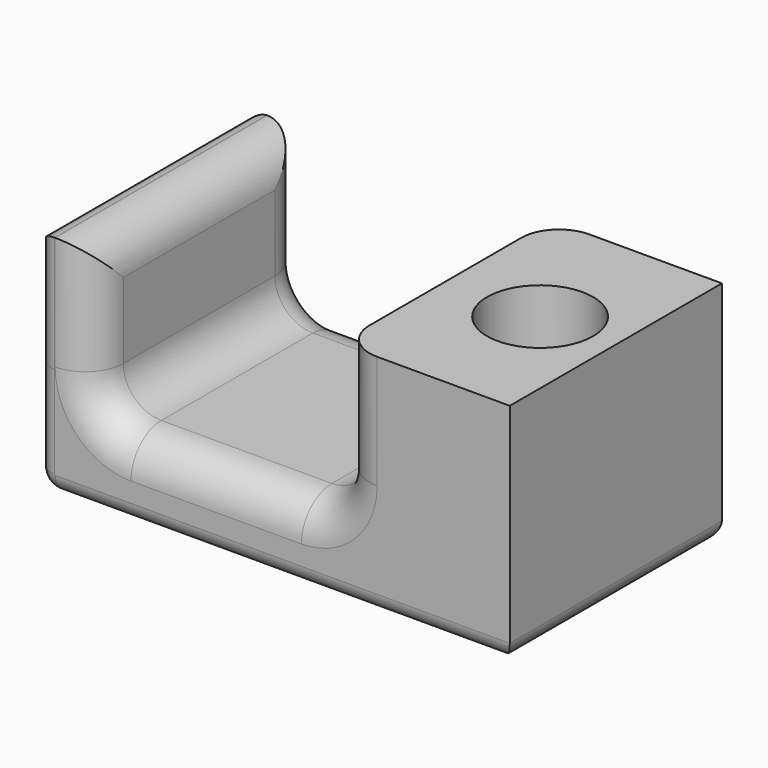
from build123d import *

# Parameters (mm, degrees)
F0_W         = 1.5
F0_H         = 7
F0_W_2       = 6.5
F0_W_3       = 4.5
F0_R         = 1.4
F1_DEPTH     = 2
F2_DEPTH     = 4
F3_F1_R      = 1
F3_F2_R      = 1
F4_T1_DEPTH  = 5.9980686292
F4_T3_DEPTH  = 13.2514489274
F4_T5_DEPTH  = 9.5048292256
F4_T7_DEPTH  = 2.4368940733
F4_T9_DEPTH  = 4.3169803418
F4_T11_DEPTH = 9.509680201
F4_T13_DEPTH = 4.2548401974
F4_T15_DEPTH = 2.4990342177
F4_S19_W     = 0.551502254
F4_S19_H     = 0.5515022539
F4_T20_DEPTH = 0.551502254
F4_S25_W     = 0.551502254
F4_S25_H     = 0.5515022539
F4_T26_DEPTH = 0.551502254


# Not quite as in the source:
# - a fillet or chamfer that OpenCascade refuses, or shapes differently, is made with other operations: its cross-section is extruded or revolved along the edge and cut away or added


with BuildPart() as f1:
    # F0 (on Top) → F1 (new body)
    with BuildSketch(Plane.XY):
        with Locations((-7.4809225276, 0.9873391916)):
            Rectangle(F0_W, F0_H)
        with Locations((-3.4809225276, 0.9873391916)):
            Rectangle(F0_W_2, F0_H)
        with Locations((2.0190774724, 0.9873391916)):
            Rectangle(F0_W_3, F0_H)
        with Locations((2.2690774724, 0.9873391916)):
            Circle(F0_R, mode=Mode.SUBTRACT)
    extrude(amount=-F1_DEPTH)

    # F0 (on Top) → F2 (join)
    with BuildSketch(Plane.XY):
        with Locations((-7.4809225276, 0.9873391916)):
            Rectangle(F0_W, F0_H)
        with Locations((2.0190774724, 0.9873391916)):
            Rectangle(F0_W_3, F0_H)
        with Locations((2.2690774724, 0.9873391916)):
            Circle(F0_R, mode=Mode.SUBTRACT)
    extrude(amount=F2_DEPTH)

    # F3: fillet of radius 1 on 7 edges, made by hand

    # F3_f1
    f3_f1_edges = [f1.edges().sort_by_distance(p)[0] for p in [
        (-0.2309225276, 0.9873391916, 0),
        (-6.7309225276, 0.9873391916, 0),
    ]]
    fillet(f3_f1_edges, radius=F3_F1_R)

    # F3_f2
    f3_f2_edges = [f1.edges().sort_by_distance(p)[0] for p in [
        (-3.4809225276, 4.4873391916, 0),
        (-3.4809225276, -2.5126608084, 0),
        (-6.7309225276, -2.5126608084, 2.5),
        (-6.7309225276, 4.4873391916, 2.5),
        (-6.7309225276, 0.9873391916, 4),
        (-6.4380293088, 4.4873391916, 0.2928932188),
        (-6.4380293088, -2.5126608084, 0.2928932188),
        (-0.5238157464, -2.5126608084, 0.2928932188),
        (-0.5238157464, 4.4873391916, 0.2928932188),
    ]]
    fillet(f3_f2_edges, radius=F3_F2_R)

    # F4: fillet of radius 0.5 on 8 edges, made by hand

    # F4_s2 → F4_t1 (cut)
    with BuildSketch(Plane.XZ.offset(-3.9863735062)):
        with BuildLine():
            ThreePointArc((-8.2313225276, -1.4990343146), (-8.0844759182, -1.8535533906), (-7.7299568422, -2.0004))
            Line((-7.7299568422, -2.0004), (-7.7299568422, -2.0505365685))
            ThreePointArc((-7.7299568422, -2.0505365685), (-7.9804396849, -2.0501365685), (-8.2309225276, -2.0501365685))
            Line((-8.2309225276, -2.0501365685), (-8.2810590962, -2))
            ThreePointArc((-8.2810590962, -2), (-8.2810590962, -1.7495171573), (-8.2814590962, -1.4990343146))
            Line((-8.2814590962, -1.4990343146), (-8.2313225276, -1.4990343146))
        make_face()
    extrude(amount=F4_T1_DEPTH, mode=Mode.SUBTRACT)

    # F4_s4 → F4_t3 (cut)
    with BuildSketch(Plane.YZ.offset(-7.7299568422)):
        with BuildLine():
            ThreePointArc((-2.011695123, -2.0004), (-2.366214199, -1.8535533906), (-2.5130608084, -1.4990343146))
            Line((-2.5130608084, -1.4990343146), (-2.563197377, -1.4990343146))
            ThreePointArc((-2.563197377, -1.4990343146), (-2.562797377, -1.7495171573), (-2.562797377, -2))
            Line((-2.562797377, -2), (-2.5126608084, -2.0501365685))
            ThreePointArc((-2.5126608084, -2.0501365685), (-2.2621779657, -2.0501365685), (-2.011695123, -2.0505365685))
            Line((-2.011695123, -2.0505365685), (-2.011695123, -2.0004))
        make_face()
        with BuildLine():
            ThreePointArc((4.4877391916, -1.4990343146), (4.3408925822, -1.8535533906), (3.9863735062, -2.0004))
            Line((3.9863735062, -2.0004), (3.9863735062, -2.0505365685))
            ThreePointArc((3.9863735062, -2.0505365685), (4.2368563489, -2.0501365685), (4.4873391916, -2.0501365685))
            Line((4.4873391916, -2.0501365685), (4.5374757601, -2))
            ThreePointArc((4.5374757601, -2), (4.5374757601, -1.7495171573), (4.5378757601, -1.4990343146))
            Line((4.5378757601, -1.4990343146), (4.4877391916, -1.4990343146))
        make_face()
    extrude(amount=F4_T3_DEPTH, mode=Mode.SUBTRACT)

    # F4_s6 → F4_t5 (cut)
    with BuildSketch(Plane.XZ.offset(-5.7397538044)):
        with BuildLine():
            ThreePointArc((3.768111787, -2.0004), (4.122630863, -1.8535533906), (4.2694774724, -1.4990343146))
            Line((4.2694774724, -1.4990343146), (4.3196140409, -1.4990343146))
            ThreePointArc((4.3196140409, -1.4990343146), (4.3192140409, -1.7495171573), (4.3192140409, -2))
            Line((4.3192140409, -2), (4.2690774724, -2.0501365685))
            ThreePointArc((4.2690774724, -2.0501365685), (4.0185946297, -2.0501365685), (3.768111787, -2.0505365685))
            Line((3.768111787, -2.0505365685), (3.768111787, -2.0004))
        make_face()
    extrude(amount=F4_T5_DEPTH, mode=Mode.SUBTRACT)

    # F4_s8 → F4_t7 (cut)
    with BuildSketch(Plane.XY.offset(-1.4990343146)):
        with BuildLine():
            ThreePointArc((-8.2313225276, -2.011695123), (-8.0844759182, -2.366214199), (-7.7299568422, -2.5130608084))
            Line((-7.7299568422, -2.5130608084), (-7.7299568422, -2.563197377))
            ThreePointArc((-7.7299568422, -2.563197377), (-7.9804396849, -2.562797377), (-8.2309225276, -2.562797377))
            Line((-8.2309225276, -2.562797377), (-8.2810590962, -2.5126608084))
            ThreePointArc((-8.2810590962, -2.5126608084), (-8.2810590962, -2.2621779657), (-8.2814590962, -2.011695123))
            Line((-8.2814590962, -2.011695123), (-8.2313225276, -2.011695123))
        make_face()
    extrude(amount=F4_T7_DEPTH, mode=Mode.SUBTRACT)

    # F4_s10 → F4_t9 (cut)
    with BuildSketch(Plane.XY.offset(0.9378597587)):
        with BuildLine():
            ThreePointArc((-8.2313225276, -2.0116941886), (-8.0841327357, -2.3665561153), (-7.7289866453, -2.5130589353))
            Line((-7.7289866453, -2.5130589353), (-7.7288896256, -2.56319541))
            ThreePointArc((-7.7288896256, -2.56319541), (-7.7309225276, -2.562797377), (-8.2309225276, -2.562797377))
            Line((-8.2309225276, -2.562797377), (-8.2810590962, -2.5126608084))
            ThreePointArc((-8.2810590962, -2.5126608084), (-8.2810590962, -2.2621774985), (-8.2814590962, -2.0116941886))
            Line((-8.2814590962, -2.0116941886), (-8.2313225276, -2.0116941886))
        make_face()
    extrude(amount=F4_T9_DEPTH, mode=Mode.SUBTRACT)

    # F4_s12 → F4_t11 (cut)
    with BuildSketch(Plane.XZ.offset(-5.7421792921)):
        with BuildLine():
            ThreePointArc((-7.7289866453, 4.0003981269), (-8.0841327357, 3.8538953069), (-8.2313225276, 3.4990333802))
            Line((-8.2313225276, 3.4990333802), (-8.2814590962, 3.4990333802))
            ThreePointArc((-8.2814590962, 3.4990333802), (-8.2810590962, 3.7495166901), (-8.2810590962, 4))
            Line((-8.2810590962, 4), (-8.2309225276, 4.0501365685))
            ThreePointArc((-8.2309225276, 4.0501365685), (-7.7309225276, 4.0501365685), (-7.7288896256, 4.0505346016))
            Line((-7.7288896256, 4.0505346016), (-7.7289866453, 4.0003981269))
        make_face()
    extrude(amount=F4_T11_DEPTH, mode=Mode.SUBTRACT)

    # F4_s14 → F4_t13 (cut)
    with BuildSketch(Plane.XY.offset(0.9999999031)):
        with BuildLine():
            ThreePointArc((-7.7289866453, 4.4877373185), (-8.0841327357, 4.3412344984), (-8.2313225276, 3.9863725718))
            Line((-8.2313225276, 3.9863725718), (-8.2814590962, 3.9863725718))
            ThreePointArc((-8.2814590962, 3.9863725718), (-8.2810590962, 4.2368558817), (-8.2810590962, 4.4873391916))
            Line((-8.2810590962, 4.4873391916), (-8.2309225276, 4.5374757601))
            ThreePointArc((-8.2309225276, 4.5374757601), (-7.7309225276, 4.5374757601), (-7.7288896256, 4.5378737932))
            Line((-7.7288896256, 4.5378737932), (-7.7289866453, 4.4877373185))
        make_face()
    extrude(amount=F4_T13_DEPTH, mode=Mode.SUBTRACT)

    # F4_s16 → F4_t15 (cut)
    with BuildSketch(Plane.XY.offset(-1.4990343146)):
        with BuildLine():
            ThreePointArc((-7.7299568422, 4.4877391916), (-8.0844759182, 4.3408925822), (-8.2313225276, 3.9863735062))
            Line((-8.2313225276, 3.9863735062), (-8.2814590962, 3.9863735062))
            ThreePointArc((-8.2814590962, 3.9863735062), (-8.2810590962, 4.2368563489), (-8.2810590962, 4.4873391916))
            Line((-8.2810590962, 4.4873391916), (-8.2309225276, 4.5374757601))
            ThreePointArc((-8.2309225276, 4.5374757601), (-7.9804396849, 4.5374757601), (-7.7299568422, 4.5378757601))
            Line((-7.7299568422, 4.5378757601), (-7.7299568422, 4.4877391916))
        make_face()
    extrude(amount=F4_T15_DEPTH, mode=Mode.SUBTRACT)


with BuildPart() as f4_tool18:
    # F4_s19 → F4_t20 (new body)
    with BuildSketch(Plane.XZ.offset(-3.9863735062)):
        with Locations((-8.0057079692, -1.7747854416)):
            Rectangle(F4_S19_W, F4_S19_H)
    extrude(amount=-F4_T20_DEPTH)

    # F4_s21 → F4_t22 (revolve, cut)
    with BuildSketch(Plane(origin=(-7.7299568422, 3.9863735062, -1.4990343146), x_dir=(0.7071067812, 0, 0.7071067812), z_dir=(-0.7071067812, 0, 0.7071067812))):
        with BuildLine():
            ThreePointArc((0, -0.5013656854), (0.5013656854, 0), (0, 0.5013656854))
            Line((0, 0.5013656854), (0, -0.5013656854))
        make_face()
    revolve(axis=Axis((-7.7299568422, 3.9863735062, -1.4990343146), (0, 1, 0)), mode=Mode.SUBTRACT)


with BuildPart() as f1_1:
    add(f1.part)

    # F4_t17: cut F4_tool18
    add(f4_tool18.part, mode=Mode.SUBTRACT)


with BuildPart() as f4_tool24:
    # F4_s25 → F4_t26 (new body)
    with BuildSketch(Plane.YZ.offset(-7.7299568422)):
        with Locations((-2.28744625, -1.7747854416)):
            Rectangle(F4_S25_W, F4_S25_H)
    extrude(amount=-F4_T26_DEPTH)

    # F4_s27 → F4_t28 (revolve, cut)
    with BuildSketch(Plane(origin=(-7.7299568422, -2.011695123, -1.4990343146), x_dir=(0, 0.7071067812, 0.7071067812), z_dir=(0, -0.7071067812, 0.7071067812))):
        with BuildLine():
            ThreePointArc((0, -0.5013656854), (0.5013656854, 0), (0, 0.5013656854))
            Line((0, 0.5013656854), (0, -0.5013656854))
        make_face()
    revolve(axis=Axis((-7.7299568422, -2.011695123, -1.4990343146), (-1, 0, 0)), mode=Mode.SUBTRACT)


with BuildPart() as f1_2:
    add(f1_1.part)

    # F4_t23: cut F4_tool24
    add(f4_tool24.part, mode=Mode.SUBTRACT)

    # F4_s29 → F4_t30 (revolve, cut)
    with BuildSketch(Plane.XZ.offset(-0.9873391916)):
        with BuildLine():
            ThreePointArc((4.1700431578, -2.0004), (3.8155240818, -1.8535533906), (3.6686774724, -1.4990343146))
            Line((3.6686774724, -1.4990343146), (3.6185409038, -1.4990343146))
            ThreePointArc((3.6185409038, -1.4990343146), (3.6189409038, -1.7495171573), (3.6189409038, -2))
            Line((3.6189409038, -2), (3.6690774724, -2.0501365685))
            ThreePointArc((3.6690774724, -2.0501365685), (3.9195603151, -2.0501365685), (4.1700431578, -2.0505365685))
            Line((4.1700431578, -2.0505365685), (4.1700431578, -2.0004))
        make_face()
    revolve(axis=Axis((2.2690774724, 0.9873391916, -2), (0, 0, 1)), mode=Mode.SUBTRACT)


solid = f1_2.part
